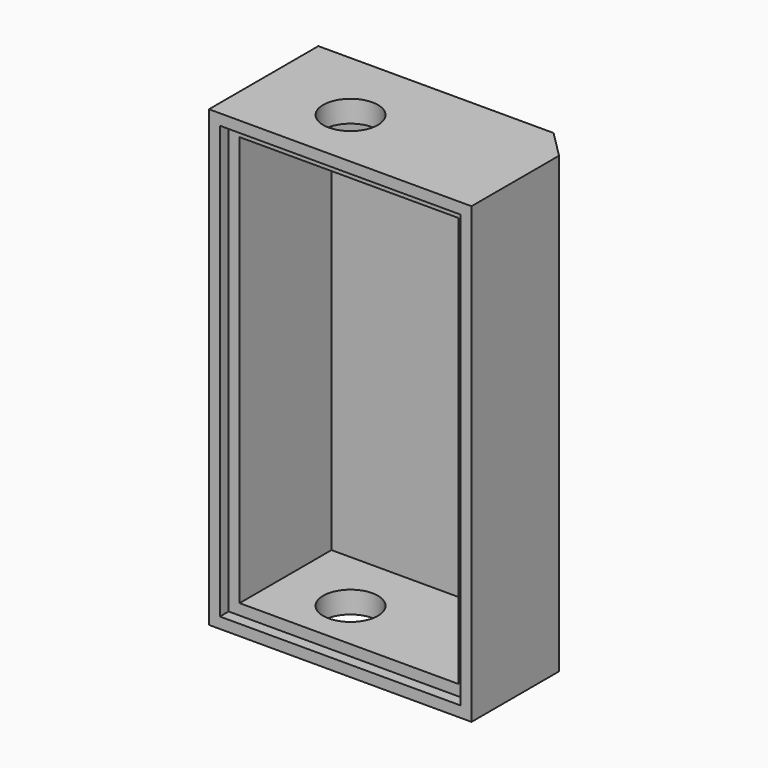
from build123d import *

# Parameters (mm, degrees)
F0_W     = 48
F0_H     = 83
F0_W_2   = 44
F0_H_2   = 79
F0_W_3   = 40
F0_H_3   = 75
F1_DEPTH = 2
F2_DEPTH = 25
F3_DEPTH = 23
F4_SIZE2 = 5
F4_SIZE  = 5
F6_DEPTH = 2
F12_D    = 10


with BuildPart() as f1:
    # F0 (on Front) → F1 (new body)
    with BuildSketch(Plane.XZ):
        Rectangle(F0_W, F0_H)
        Rectangle(F0_W_2, F0_H_2, mode=Mode.SUBTRACT)
        Rectangle(F0_W_2, F0_H_2)
        Rectangle(F0_W_3, F0_H_3, mode=Mode.SUBTRACT)
        Rectangle(F0_W_3, F0_H_3)
    extrude(amount=F1_DEPTH)

    # F0 (on Front) → F2 (join)
    with BuildSketch(Plane.XZ):
        Rectangle(F0_W, F0_H)
        Rectangle(F0_W_2, F0_H_2, mode=Mode.SUBTRACT)
    extrude(amount=F2_DEPTH)

    # F0 (on Front) → F3 (join)
    with BuildSketch(Plane.XZ):
        Rectangle(F0_W_2, F0_H_2)
        Rectangle(F0_W_3, F0_H_3, mode=Mode.SUBTRACT)
    extrude(amount=F3_DEPTH)

    # F4
    f4_edges = [f1.edges().sort_by_distance(p)[0] for p in [
        (24, 0, 0),
    ]]
    chamfer(f4_edges, length=F4_SIZE, length2=F4_SIZE2)

    # F6 (add): a face of the model
    f6_faces = [f1.faces().sort_by_distance(p)[0] for p in [
        (21.5, -2.5, 0),
    ]]
    extrude(f6_faces, amount=-F6_DEPTH)

    # F12 (through all)
    with Locations(Plane.XY.offset(41.5)):
        with Locations((-7.1147754788, -13.7537298724)):
            Hole(F12_D / 2)


solid = f1.part
